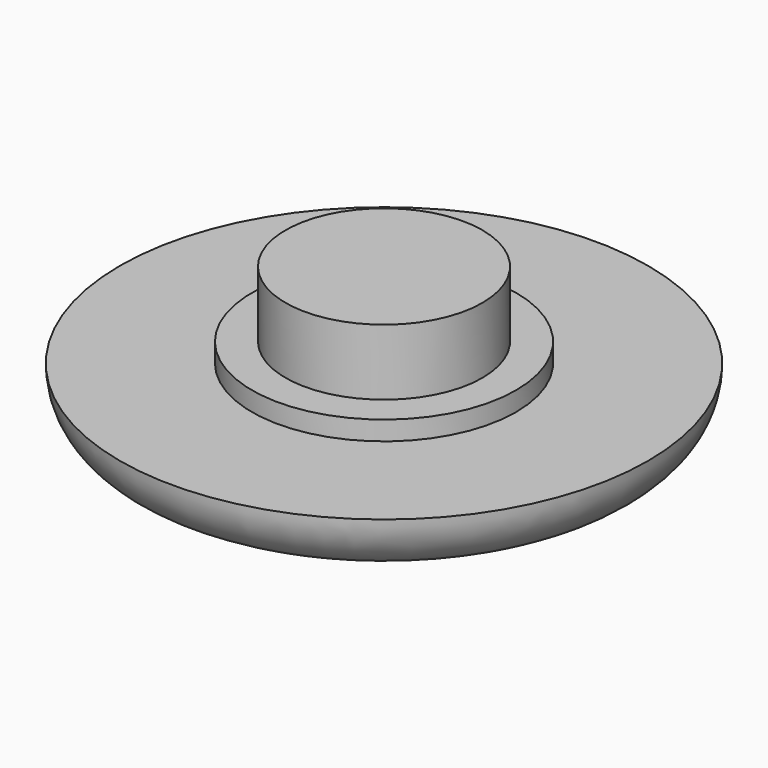
from build123d import *

# Parameters (mm, degrees)
F0_R     = 11
F0_R_2   = 5.5
F1_DEPTH = 2.5
F0_R_3   = 4.1
F2_DEPTH = 3.3
F3_DEPTH = 6.05
F4_R     = 2.49999


# Not quite as in the source:
# - a fillet or chamfer is up to 0.001 mm smaller than in the source, because OpenCascade refuses the exact size


with BuildPart() as f1:
    # F0 (on Top) → F1 (new body)
    with BuildSketch(Plane.XY):
        Circle(F0_R)
        Circle(F0_R_2, mode=Mode.SUBTRACT)
    extrude(amount=F1_DEPTH)

    # F0 (on Top) → F2 (join, through all)
    with BuildSketch(Plane.XY):
        Circle(F0_R_2)
        Circle(F0_R_3, mode=Mode.SUBTRACT)
    extrude(amount=F2_DEPTH)

    # F0 (on Top) → F3 (join, through all)
    with BuildSketch(Plane.XY):
        Circle(F0_R_3)
    extrude(amount=F3_DEPTH)

    # F4 (radius 2.5 in the source; OpenCascade refuses exactly that, so slightly less here)
    f4_edges = [f1.edges().sort_by_distance(p)[0] for p in [
        (-11, 0, 0),
    ]]
    fillet(f4_edges, radius=F4_R)


solid = f1.part
